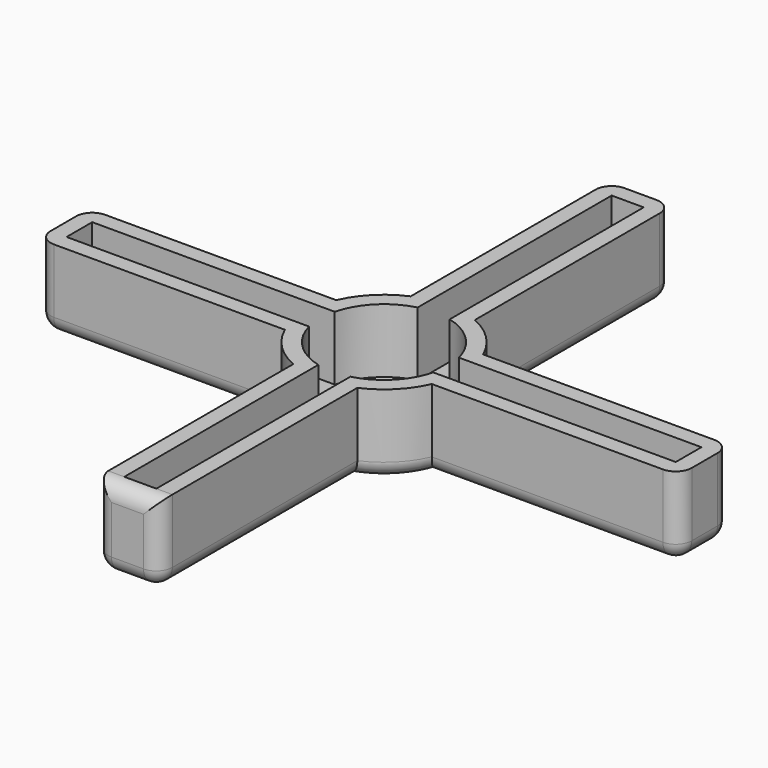
from build123d import *

# Parameters (mm, degrees)
F0_W     = 4
F0_H     = 4
F1_DEPTH = 5
F2_T     = -1
F3_R     = 0.99999


# Not quite as in the source:
# - a fillet or chamfer is up to 0.001 mm smaller than in the source, because OpenCascade refuses the exact size


with BuildPart() as f1:
    # F0 (on Top) → F1 (new body)
    with BuildSketch(Plane.XY):
        with BuildLine():
            ThreePointArc((-2, 4.582575695), (0, 5), (2, 4.582575695))
            Line((2, 4.582575695), (2, 20))
            Line((2, 20), (-2, 20))
            Line((-2, 20), (-2, 4.582575695))
        make_face()
        with BuildLine():
            Line((2, 2), (2, 4.582575695))
            ThreePointArc((2, 4.582575695), (0, 5), (-2, 4.582575695))
            Line((-2, 4.582575695), (-2, 2))
            Line((-2, 2), (2, 2))
        make_face()
        Rectangle(F0_W, F0_H)
        with BuildLine():
            ThreePointArc((-2, -4.582575695), (0, -5), (2, -4.582575695))
            Line((2, -4.582575695), (2, -2))
            Line((2, -2), (-2, -2))
            Line((-2, -2), (-2, -4.582575695))
        make_face()
        with BuildLine():
            Line((2, -20), (2, -4.582575695))
            ThreePointArc((2, -4.582575695), (0, -5), (-2, -4.582575695))
            Line((-2, -4.582575695), (-2, -20))
            Line((-2, -20), (2, -20))
        make_face()
        with BuildLine():
            ThreePointArc((4.582575695, 2), (4.8945315647, 1.0215482184), (5, 0))
            ThreePointArc((5, 0), (4.8945315647, -1.0215482184), (4.582575695, -2))
            Line((4.582575695, -2), (20, -2))
            Line((20, -2), (20, 2))
            Line((20, 2), (4.582575695, 2))
        make_face()
        with BuildLine():
            Line((2, 2), (4.582575695, 2))
            ThreePointArc((4.582575695, 2), (3.5355339059, 3.5355339059), (2, 4.582575695))
            Line((2, 4.582575695), (2, 2))
        make_face()
        with BuildLine():
            ThreePointArc((4.582575695, -2), (4.8945315647, -1.0215482184), (5, 0))
            ThreePointArc((5, 0), (4.8945315647, 1.0215482184), (4.582575695, 2))
            Line((4.582575695, 2), (2, 2))
            Line((2, 2), (2, -2))
            Line((2, -2), (4.582575695, -2))
        make_face()
        with BuildLine():
            ThreePointArc((2, -4.582575695), (3.5355339059, -3.5355339059), (4.582575695, -2))
            Line((4.582575695, -2), (2, -2))
            Line((2, -2), (2, -4.582575695))
        make_face()
        with BuildLine():
            Line((-2, -2), (-2, 2))
            Line((-2, 2), (-4.582575695, 2))
            ThreePointArc((-4.582575695, 2), (-5, 0), (-4.582575695, -2))
            Line((-4.582575695, -2), (-2, -2))
        make_face()
        with BuildLine():
            Line((-2, 2), (-2, 4.582575695))
            ThreePointArc((-2, 4.582575695), (-3.5355339059, 3.5355339059), (-4.582575695, 2))
            Line((-4.582575695, 2), (-2, 2))
        make_face()
        with BuildLine():
            ThreePointArc((-4.582575695, -2), (-3.5355339059, -3.5355339059), (-2, -4.582575695))
            Line((-2, -4.582575695), (-2, -2))
            Line((-2, -2), (-4.582575695, -2))
        make_face()
        with BuildLine():
            ThreePointArc((-4.582575695, -2), (-5, 0), (-4.582575695, 2))
            Line((-4.582575695, 2), (-20, 2))
            Line((-20, 2), (-20, -2))
            Line((-20, -2), (-4.582575695, -2))
        make_face()
    extrude(amount=F1_DEPTH)

    # F2
    f2_openings = [f1.faces().sort_by_distance(p)[0] for p in [
        (0, 0, 5),
    ]]
    offset(amount=F2_T, openings=f2_openings, kind=Kind.INTERSECTION)

    # F3 (radius 1 in the source; OpenCascade refuses exactly that, so slightly less here)
    f3_edges = [f1.edges().sort_by_distance(p)[0] for p in [
        (0, 20, 0),
        (-2, 12.291288, 0),
        (-3.535534, 3.535534, 0),
        (-12.291288, 2, 0),
        (-20, 0, 0),
        (-12.291288, -2, 0),
        (-3.535534, -3.535534, 0),
        (-2, -12.291288, 0),
        (0, -20, 0),
        (2, -12.291288, 0),
        (3.535534, -3.535534, 0),
        (12.291288, -2, 0),
        (20, 0, 0),
        (12.291288, 2, 0),
        (3.535534, 3.535534, 0),
        (2, 12.291288, 0),
        (2, -20, 2.5),
        (-2, -20, 2.5),
        (0, -20, 5),
        (-20, 2, 2.5),
        (-20, -2, 2.5),
        (-2, 20, 2.5),
        (2, 20, 2.5),
        (20, 2, 2.5),
        (20, -2, 2.5),
    ]]
    fillet(f3_edges, radius=F3_R)


solid = f1.part
